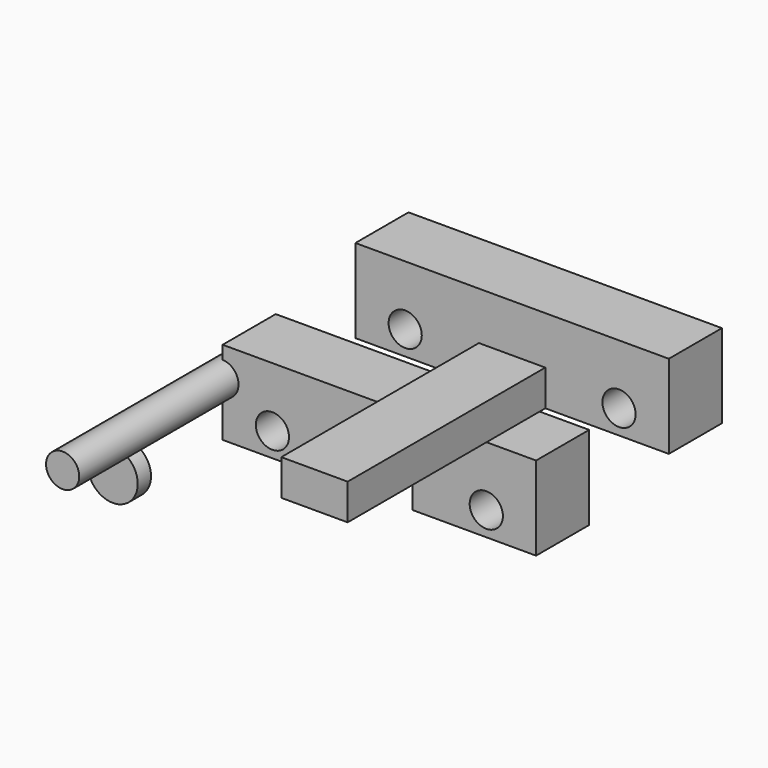
from build123d import *

# Parameters (mm, degrees)
F0_R     = 3.175
F1_DEPTH = 12.7
F3_W     = 12.7
F3_H     = 6.858
F4_DEPTH = 59.9694
F6_R     = 3.175
F7_DEPTH = 50.8
F8_R     = 4.7625
F9_DEPTH = 3.175


# Not quite as in the source:
# - a feature of the source that left no trace in its solid (it failed there, or was rolled back) is left out


with BuildPart() as f1:
    # F0 (on Front) → F1 (new body)
    with BuildSketch(Plane.XZ):
        Polygon((42.1162071086, 21.6844746424), (-17.8531928914, 21.6844746424), (-17.8531928914, 5.6570746424), (5.7815071086, 5.6570746424), (5.7815071086, 12.5150746424), (18.4815071086, 12.5150746424), (18.4815071086, 5.6570746424), (42.1162071086, 5.6570746424), align=None)
        with Locations((-8.3281928914, 10.2544746424)):
            Circle(F0_R, mode=Mode.SUBTRACT)
        with Locations((32.5912071086, 10.2544746424)):
            Circle(F0_R, mode=Mode.SUBTRACT)
    extrude(amount=F1_DEPTH)


with BuildPart() as f2_1:
    # F2: copy of F1
    add(f1.part.moved(Location((25.4, 0, 25.4))))

    # F3 (on face) → F4 (join)
    with BuildSketch(Plane(origin=(0, 0, 0), x_dir=(-1, 0, 0), z_dir=(0, 1, 0))):
        with Locations((-37.5315071086, 34.4860746424)):
            Rectangle(F3_W, F3_H)
    extrude(amount=-F4_DEPTH)


with BuildPart() as f7:
    # F6 (on Front) → F7 (new body)
    with BuildSketch(Plane.XZ):
        with Locations((-17.9878603667, 15.973219648)):
            Circle(F6_R)
    extrude(amount=F7_DEPTH)


with BuildPart() as f9:
    # F8 (on Front) → F9 (new body)
    with BuildSketch(Plane.XZ):
        with Locations((-46.4806295931, -13.3829684928)):
            Circle(F8_R)
    extrude(amount=F9_DEPTH)


solid = Compound([f1.part, f2_1.part, f7.part, f9.part])
